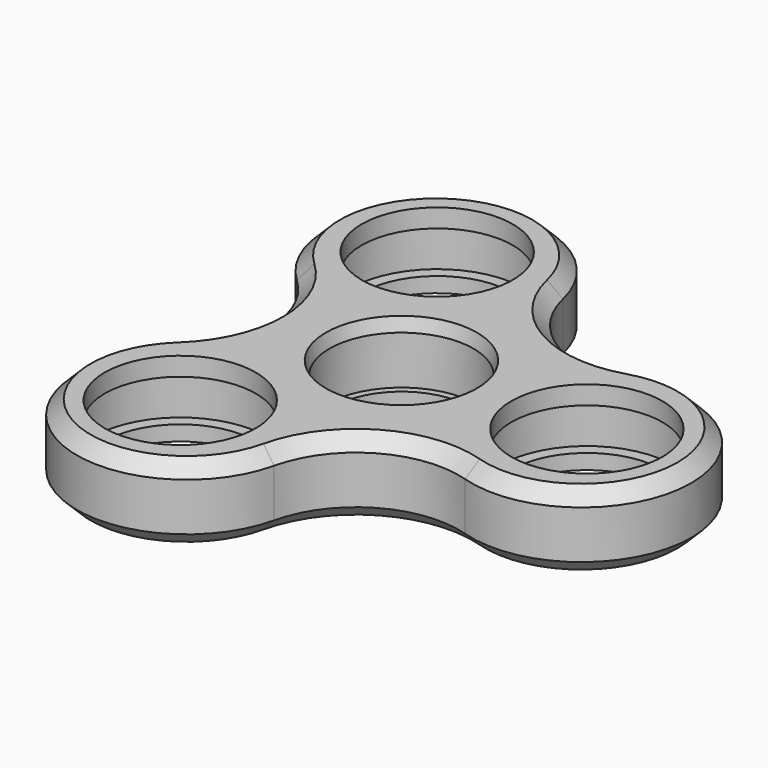
from build123d import *

# Parameters (mm, degrees)
F1_DEPTH        = 11
F5_COPIES_COUNT = 3
F6_SIZE         = 2
F7_SIZE         = 2


# Not quite as in the source:
# - a pattern or mirror of a feature is missing from the dataset's text; its kind, count and spacing are read off the source's solid


with BuildPart() as f1:
    # F0 (on Top) → F1 (new body)
    with BuildSketch(Plane.XY):
        with BuildLine():
            ThreePointArc((2.4931063701, -26.2757839441), (9.6114548877, -16.6475282001), (21.5089432149, -15.2969854229))
            ThreePointArc((21.5089432149, -15.2969854229), (42.1995974306, 0), (21.5089432149, 15.2969854229))
            ThreePointArc((21.5089432149, 15.2969854229), (9.6114548877, 16.6475282001), (2.4931063701, 26.2757839441))
            ThreePointArc((2.4931063701, 26.2757839441), (-21.0997987153, 36.5459234044), (-24.002049585, 10.9787985212))
            ThreePointArc((-24.002049585, 10.9787985212), (-19.2229097754, 0), (-24.002049585, -10.9787985212))
            ThreePointArc((-24.002049585, -10.9787985212), (-21.0997987153, -36.5459234044), (2.4931063701, -26.2757839441))
        make_face()
    extrude(amount=F1_DEPTH)

    # F2 (on Right) → F3 (revolve, cut)
    with BuildSketch(Plane.YZ):
        Polygon((0, 11), (0, 0), (10, 0), (10, 1.8), (11, 1.8), (11, 9.1), (10.5, 9.1), (11, 11), align=None)
    revolve(axis=Axis((0, 0, 3.7751235068), (0, 0, -1)), mode=Mode.SUBTRACT)

    # F4 (on Front) → F5 (revolve, cut)
    with BuildSketch(Plane.XZ):
        Polygon((16, 0), (27, 0), (27, 11), (16, 11), (16, 8.3), (14.3, 8.3), (14.3, 2.2), (16, 2.2), align=None)
    f5 = revolve(axis=Axis((27, 0, 6.29213918), (0, 0, -1)), mode=Mode.SUBTRACT)

    # F5_copies: F5 ×3 about axis
    f5_copies_axis = Axis((0, 0, 0), (0, 0, 1))
    for i in range(1, F5_COPIES_COUNT):
        add(f5.rotate(f5_copies_axis, i * 360 / F5_COPIES_COUNT), mode=Mode.SUBTRACT)

    # F6
    f6_edges = [f1.edges().sort_by_distance(p)[0] for p in [
        (9.611455, -16.647528, 11),
    ]]
    chamfer(f6_edges, length=F6_SIZE)

    # F7
    f7_edges = [f1.edges().sort_by_distance(p)[0] for p in [
        (9.611455, -16.647528, 0),
        (-21.099799, -36.545923, 0),
        (-19.22291, 0, 0),
        (-21.099799, 36.545923, 0),
        (42.199597, 0, 0),
        (9.611455, 16.647528, 0),
    ]]
    chamfer(f7_edges, length=F7_SIZE)


solid = f1.part
